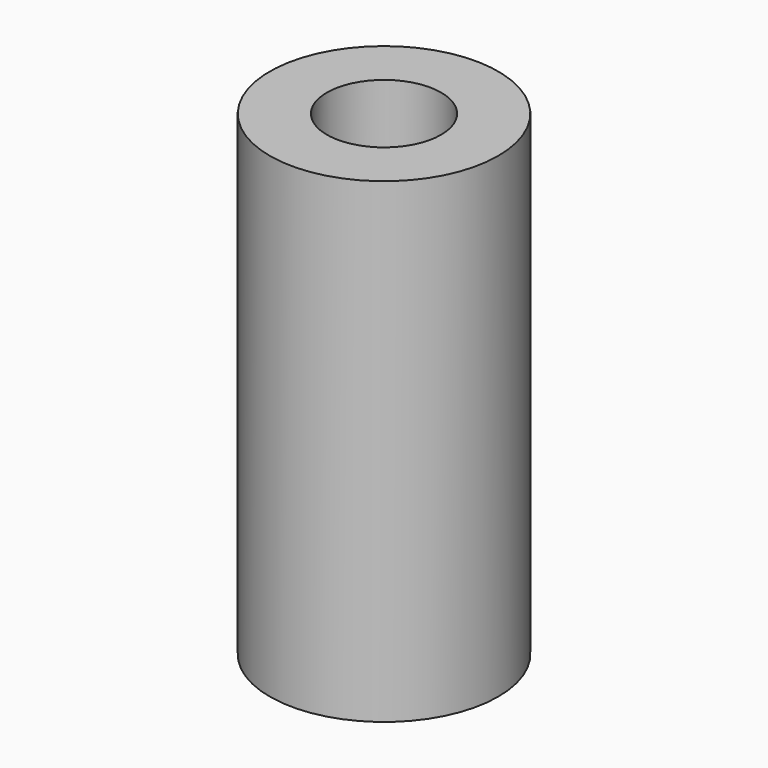
from build123d import *

# Parameters (mm, degrees)
F0_R     = 6
F0_R_2   = 4
F1_DEPTH = 13
F0_R_3   = 3
F2_DEPTH = 12
F3_SIZE  = 0.99999
F4_SIZE  = 0.5


# Not quite as in the source:
# - a fillet or chamfer is up to 0.001 mm smaller than in the source, because OpenCascade refuses the exact size


with BuildPart() as f1:
    # F0 (on Top) → F1 (new body)
    with BuildSketch(Plane.XY):
        Circle(F0_R)
        Circle(F0_R_2, mode=Mode.SUBTRACT)
    extrude(amount=-F1_DEPTH)

    # F0 (on Top) → F2 (join)
    with BuildSketch(Plane.XY):
        Circle(F0_R)
        Circle(F0_R_2, mode=Mode.SUBTRACT)
        Circle(F0_R_2)
        Circle(F0_R_3, mode=Mode.SUBTRACT)
    extrude(amount=F2_DEPTH)

    # F3 (size 1 in the source; OpenCascade refuses exactly that, so slightly less here)
    f3_edges = [f1.edges().sort_by_distance(p)[0] for p in [
        (-3, 0, 0),
    ]]
    chamfer(f3_edges, length=F3_SIZE)

    # F4
    f4_edges = [f1.edges().sort_by_distance(p)[0] for p in [
        (-4, 0, -13),
    ]]
    chamfer(f4_edges, length=F4_SIZE)


solid = f1.part
